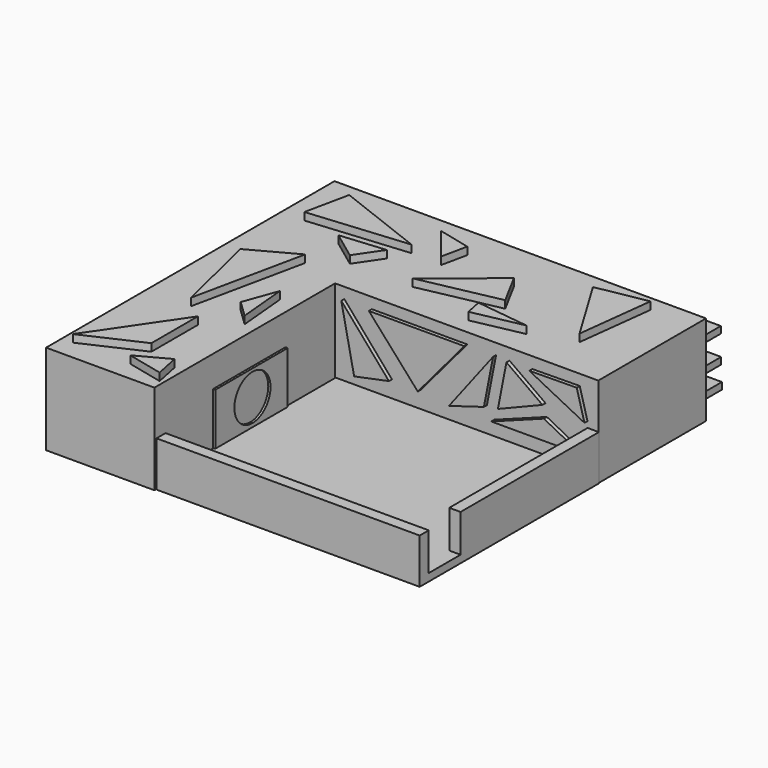
from build123d import *

# Parameters (mm, degrees)
F0_W          = 125.3317967057
F0_H          = 45.4250313342
F1_DEPTH      = 30.48
F2_W          = 36.5465022624
F2_H          = 30.48
F3_DEPTH      = 76.2
F4_W          = 88.7852944434
F4_H          = 75.5707323551
F5_DEPTH      = 2.54
F7_DEPTH      = 2.54
F9_DEPTH      = 1.27
F11_DEPTH     = 1.27
F12_W         = 88.7852944434
F12_H         = 3.81
F13_DEPTH     = 12.7
F14_W         = 30.48
F14_H         = 17.78
F15_DEPTH     = 0.762
F16_R         = 7.62
F17_DEPTH     = 0.762
F18_W         = 62.484
F18_H         = 2.286
F18_W_2       = 86.36
F18_W_3       = 124.6017685359
F19_DEPTH     = 7.62
F20_TEXT_SIZE = 17.5638331307
F21_DEPTH     = 0.508


# Not quite as in the source:
# - Text() gives the source's letters only with a copy of the font that has no kerning and outlines rounded to 1/6400 em; it was checked with that copy


with BuildPart() as f1:
    # F0 (on Top) → F1 (new body)
    with BuildSketch(Plane.XY):
        with Locations((0.9291507304, 22.7125156671)):
            Rectangle(F0_W, F0_H)
    extrude(amount=F1_DEPTH)

    # F2 (on face) → F3 (join)
    with BuildSketch(Plane.XZ):
        with Locations((-43.4634964913, 15.24)):
            Rectangle(F2_W, F2_H)
    extrude(amount=F3_DEPTH)

    # F4 (on Top) → F5 (join)
    with BuildSketch(Plane.XY):
        with Locations((19.4088798016, -37.7853661776)):
            Rectangle(F4_W, F4_H)
    extrude(amount=F5_DEPTH)

    # F6 (on face) → F7 (join)
    with BuildSketch(Plane.XY.offset(30.48)):
        Polygon((-50.7241405667, 37.8582050191), (-53.8906045258, 22.9189936072), (-20.2347878367, 26.0161533952), align=None)
        Polygon((-23.4037318118, 19.5694808907), (-38.6112779379, 18.1700140238), (-29.1388890141, 11.1497808248), align=None)
        Polygon((-38.6112779379, 4.1295485571), (-53.8906045258, -4.1295485571), (-46.6638989747, -33.8622964919), align=None)
        Polygon((-30.7651348412, -16.3117162883), (-34.894682467, -27.6679750532), (-29.2181730047, -33.1220417344), align=None)
        Polygon((-38.6112779379, -41.0890057683), (-58.0201558769, -69.5828944445), (-38.6112779379, -60.7043616474), align=None)
        Polygon((-28.1904133323, -63.9499935246), (-38.6112779379, -69.5828944445), (-26.4473815847, -72.4291425713), align=None)
        Polygon((-8.0526201054, 34.316951428), (-18.9959220588, 36.9594581425), (-9.897230607, 25.6141755207), align=None)
        Polygon((12.8015996888, 27.8744511306), (-8.0526201054, 11.1497808248), (18.8523573957, 16.6805516245), align=None)
        Polygon((32.2104766965, 8.897086981), (14.2469415441, 11.1497808248), (15.4195662491, 5.4454328327), align=None)
        Polygon((49.1416268051, 40.0566197932), (32.2104766965, 36.9594581425), (46.0444651544, 14.0404645354), align=None)
    extrude(amount=F7_DEPTH)

    # F8 (on face) → F9 (join)
    with BuildSketch(Plane.XZ):
        Polygon((-6.0178312811, 8.1982673441), (-22.0930837095, 26.8420651555), (-17.7570581436, 5.7813678868), align=None)
        Polygon((19.408877939, 26.8420651555), (-12.8015996888, 26.8420651555), (3.7165926769, 8.2590971142), align=None)
        Polygon((29.1133187711, 26.8420651555), (14.2469415441, 7.4331872165), (26.0161533952, 10.943303816), align=None)
        Polygon((46.2509393692, 14.0404645354), (28.4938849509, 7.4331872165), (59.0525455773, 7.4331872165), align=None)
    extrude(amount=F9_DEPTH)

    # F10 (on face) → F11 (join)
    with BuildSketch(Plane.XZ):
        Polygon((45.7807965577, 17.9768241942), (33.6212217808, 26.6709197313), (30.7391976572, 11.8765487006), align=None)
        Polygon((57.332392782, 26.8420651555), (41.3425527513, 26.6709197313), (59.9467009306, 17.2472503036), align=None)
    extrude(amount=F11_DEPTH)

    # F12 (on face) → F13 (join)
    with BuildSketch(Plane.XY.offset(2.54)):
        with Locations((19.4088798016, -73.6657323551)):
            Rectangle(F12_W, F12_H)
        Polygon((59.9915270233, -58.3426170051), (63.8015270233, -58.3426170051), (63.8015270233, 0), (63.5950490832, 0), (59.9915270233, 0), align=None)
    extrude(amount=F13_DEPTH)

    # F14 (on face) → F15 (join)
    with BuildSketch(Plane.YZ.offset(-25.1902453601)):
        with Locations((-36.2081946805, 11.1381291161)):
            Rectangle(F14_W, F14_H)
    extrude(amount=F15_DEPTH)

    # F16 (on face) → F17 (cut)
    with BuildSketch(Plane.YZ.offset(-24.4282453601)):
        with Locations((-35.8107872307, 11.3981552422)):
            Circle(F16_R)
    extrude(amount=-F17_DEPTH, mode=Mode.SUBTRACT)

    # F18 (on face) → F19 (join)
    with BuildSketch(Plane(origin=(0, 45.4250313342, 0), x_dir=(-1, 0, 0), z_dir=(0, 1, 0))):
        with Locations((-31.242, 23.6220089166)):
            Rectangle(F18_W, F18_H)
        with Locations((-19.4310216699, 14.4780050257)):
            Rectangle(F18_W_2, F18_H)
        with Locations((-0.5641366454, 7.1120026479)):
            Rectangle(F18_W_3, F18_H)
    extrude(amount=F19_DEPTH)

    # F20 (on face) → F21 (join)
    with BuildSketch(Plane(origin=(-61.7367476225, 0, 0), x_dir=(0, -1, 0), z_dir=(-1, 0, 0))):
        with Locations((-35.3843607008, 9.6060633659)):
            Text('CONCERTO', F20_TEXT_SIZE, font='Open Sans', font_style=FontStyle.BOLD, text_align=(TextAlign.LEFT, TextAlign.BOTTOM))
    extrude(amount=F21_DEPTH)


solid = f1.part
